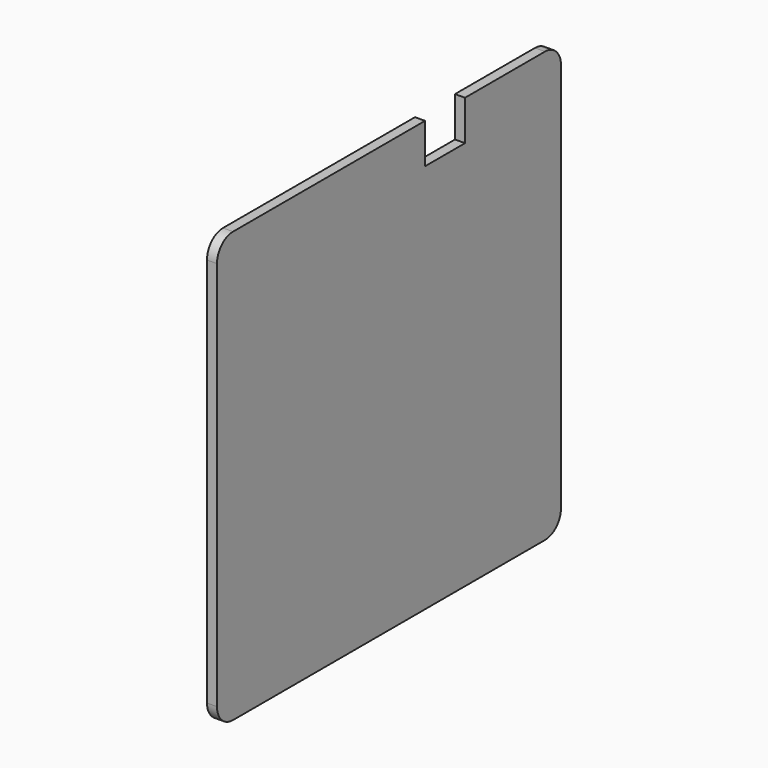
from build123d import *

# Parameters (mm, degrees)
F1_DEPTH = 1
F2_R     = 2


with BuildPart() as f1:
    # F0 (on Right) → F1 (new body)
    with BuildSketch(Plane.YZ):
        Polygon((-15.4019305557, 26.6723162987), (-15.4019305557, -16.3276837013), (27.5980694443, -16.3276837013), (27.5980694443, 26.6723162987), (15.5980694443, 26.6723162987), (15.5980694443, 22.6723162987), (10.5980694443, 22.6723162987), (10.5980694443, 26.6723162987), align=None)
    extrude(amount=F1_DEPTH)

    # F2
    f2_edges = [f1.edges().sort_by_distance(p)[0] for p in [
        (0.5, -15.401931, 26.672316),
        (0.5, -15.401931, -16.327684),
        (0.5, 27.598069, -16.327684),
        (0.5, 27.598069, 26.672316),
    ]]
    fillet(f2_edges, radius=F2_R)


solid = f1.part
